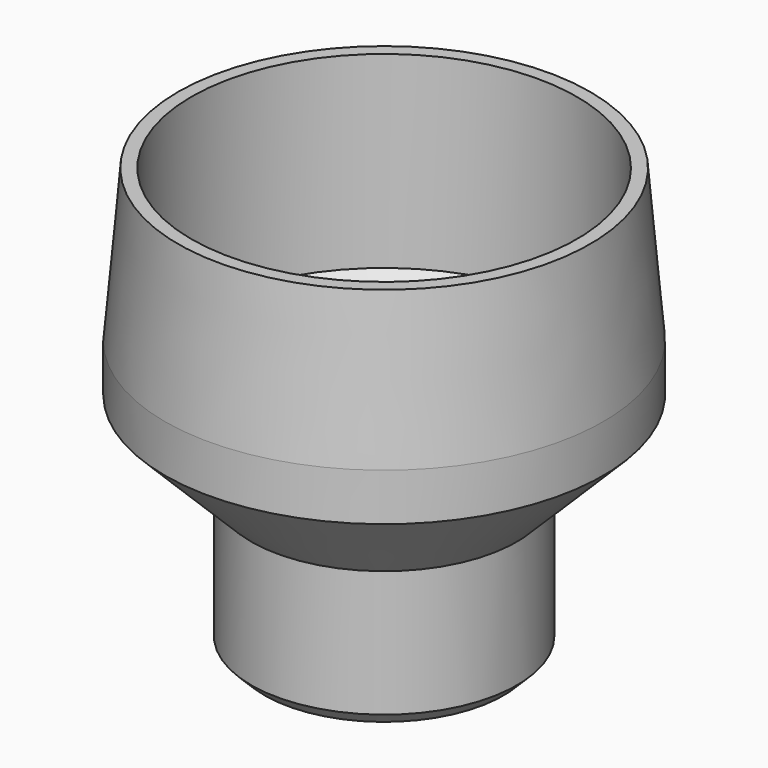
from build123d import *

# Parameters (mm, degrees)
F2_SIZE2 = 11.4300523028
F2_SIZE  = 1
F3_SIZE  = 1


# Not quite as in the source:
# - a fillet or chamfer that OpenCascade refuses, or shapes differently, is made with other operations: its cross-section is extruded or revolved along the edge and cut away or added


with BuildPart() as f1:
    # F0 (on Front) → F1 (revolve)
    with BuildSketch(Plane.XZ):
        Polygon((-14.5, 15), (-16.5, 15), (-16.5, 0), (-10, -6.5), (-10, -17), (-8, -17), (-8, -5.6715728753), (-14.5, 0.8284271247), align=None)
    revolve(axis=Axis((0, 0, 0.14814813), (0, 0, -1)))

    # F2
    f2_edges = [f1.edges().sort_by_distance(p)[0] for p in [
        (16.5, 0, 15),
    ]]
    chamfer(f2_edges, length=F2_SIZE, length2=F2_SIZE2)

    # F3
    f3_edges = [f1.edges().sort_by_distance(p)[0] for p in [
        (10, 0, -17),
    ]]
    chamfer(f3_edges, length=F3_SIZE)

    # F4: chamfer of 1 x 11.4300523028 on 1 edges, made by hand

    # F4_s1 → F4_t2 (revolve, cut)
    with BuildSketch(Plane.XZ):
        Polygon((-9, -17), (-8, -5.5699476972), (-8, -17), align=None)
    revolve(axis=Axis((0, 0, -17), (0, 0, -1)), mode=Mode.SUBTRACT)


solid = f1.part
